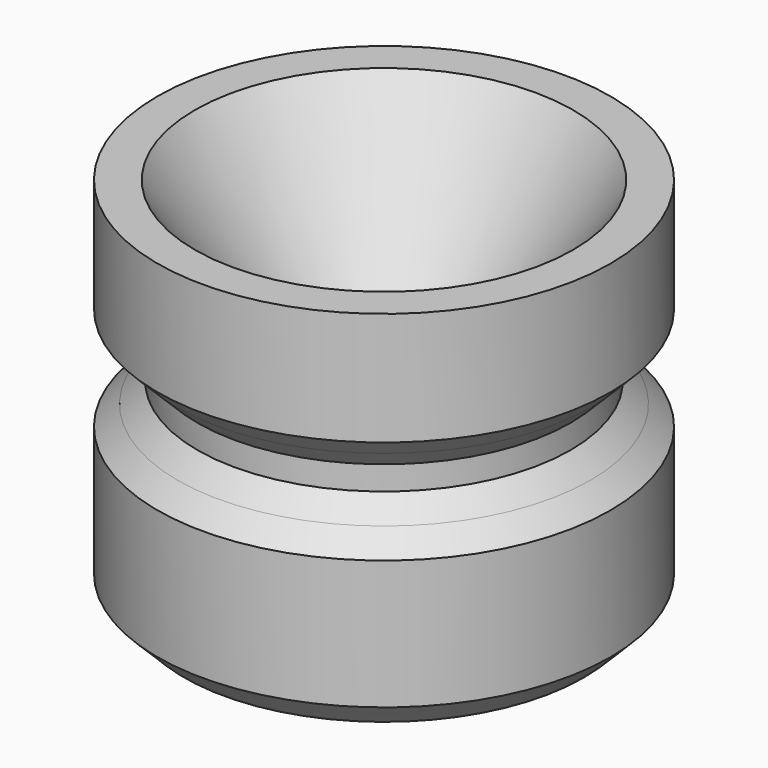
from build123d import *

# Parameters (mm, degrees)
F0_R     = 8.5
F0_R_2   = 7
F1_DEPTH = 6.6
F0_R_3   = 3.1
F2_DEPTH = 9
F3_R     = 8.5
F3_R_2   = 7
F3_R_3   = 3.1
F4_DEPTH = 5
F0_R_4   = 2.6
F5_DEPTH = 6.2
F6_SIZE  = 1
F7_SIZE2 = 4
F7_SIZE  = 6
F8_SIZE  = 0.74999


# Not quite as in the source:
# - a fillet or chamfer is up to 0.001 mm smaller than in the source, because OpenCascade refuses the exact size


with BuildPart() as f1:
    # F0 (on Top) → F1 (new body)
    with BuildSketch(Plane.XY):
        Circle(F0_R)
        Circle(F0_R_2, mode=Mode.SUBTRACT)
    extrude(amount=F1_DEPTH)

    # F0 (on Top) → F2 (join)
    with BuildSketch(Plane.XY):
        Circle(F0_R_2)
        Circle(F0_R_3, mode=Mode.SUBTRACT)
    extrude(amount=F2_DEPTH)

    # F3 (on face) → F4 (join)
    with BuildSketch(Plane.XY.offset(9)):
        Circle(F3_R)
        Circle(F3_R_2, mode=Mode.SUBTRACT)
        Circle(F3_R_2)
        Circle(F3_R_3, mode=Mode.SUBTRACT)
    extrude(amount=F4_DEPTH)

    # F0 (on Top) → F5 (join)
    with BuildSketch(Plane.XY):
        Circle(F0_R_3)
        Circle(F0_R_4, mode=Mode.SUBTRACT)
    extrude(amount=F5_DEPTH)

    # F6
    f6_edges = [f1.edges().sort_by_distance(p)[0] for p in [
        (-2.6, 0, 0),
        (-8.5, 0, 0),
    ]]
    chamfer(f6_edges, length=F6_SIZE)

    # F7
    f7_edges = [f1.edges().sort_by_distance(p)[0] for p in [
        (-3.1, 0, 14),
    ]]
    f7_side = f1.faces().sort_by_distance((-3.1, 0, 10.1))[0]
    chamfer(f7_edges, length=F7_SIZE, length2=F7_SIZE2, reference=f7_side)

    # F8 (size 0.75 in the source; OpenCascade refuses exactly that, so slightly less here)
    f8_edges = [f1.edges().sort_by_distance(p)[0] for p in [
        (-7, 0, 9),
        (-7, 0, 6.6),
        (-8.5, 0, 6.6),
        (-8.5, 0, 9),
    ]]
    chamfer(f8_edges, length=F8_SIZE)


solid = f1.part
